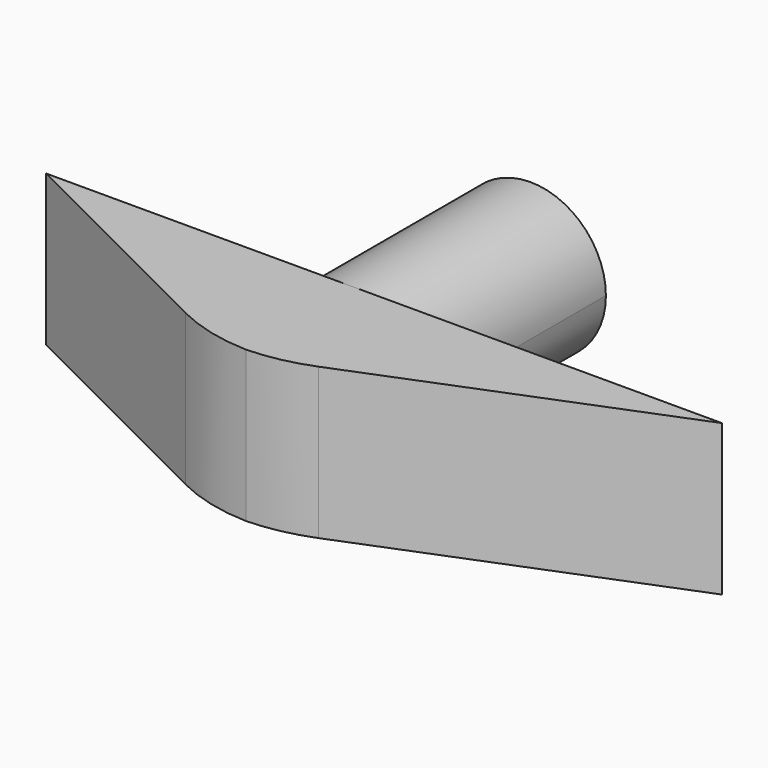
from build123d import *

# Parameters (mm, degrees)
F1_DEPTH    = 10
F2_DEPTH    = 6
F3_T1_DEPTH = 68.8558929709
F4_SIZE2    = 14.99999
F4_SIZE     = 5.99999
F5_T1_DEPTH = 16.1427191
F5_T3_DEPTH = 14.4032889904


# Not quite as in the source:
# - a fillet or chamfer that OpenCascade refuses, or shapes differently, is made with other operations: its cross-section is extruded or revolved along the edge and cut away or added
# - a fillet or chamfer is up to 0.001 mm smaller than in the source, because OpenCascade refuses the exact size


with BuildPart() as f1:
    # F0 (on Front) → F1 (new body)
    with BuildSketch(Plane.XZ):
        with BuildLine():
            ThreePointArc((2.15, -0.0081778196), (-3.4744734584, 2.4513486566), (-1.4615047685, -3.3479555451))
            Line((-1.4615047685, -3.3479555451), (-0.9384952315, -3.3479555451))
            ThreePointArc((-0.9384952315, -3.3479555451), (1.2595264762, -2.2826512779), (2.15, -0.0081778196))
        make_face()
    extrude(amount=-F1_DEPTH)


with BuildPart() as f2:
    # F0 (on Front) → F2 (new body)
    with BuildSketch(Plane.XZ):
        with BuildLine():
            Line((15.3, 3.3520444549), (-14.7, 3.3520444549))
            Line((-14.7, 3.3520444549), (-14.7, -3.3479555451))
            Line((-14.7, -3.3479555451), (-1.4615047685, -3.3479555451))
            ThreePointArc((-1.4615047685, -3.3479555451), (-3.4744734584, 2.4513486566), (2.15, -0.0081778196))
            ThreePointArc((2.15, -0.0081778196), (1.2595264762, -2.2826512779), (-0.9384952315, -3.3479555451))
            Line((-0.9384952315, -3.3479555451), (15.3, -3.3479555451))
            Line((15.3, -3.3479555451), (15.3, 3.3520444549))
        make_face()
        with BuildLine():
            ThreePointArc((2.15, -0.0081778196), (-3.4744734584, 2.4513486566), (-1.4615047685, -3.3479555451))
            Line((-1.4615047685, -3.3479555451), (-0.9384952315, -3.3479555451))
            ThreePointArc((-0.9384952315, -3.3479555451), (1.2595264762, -2.2826512779), (2.15, -0.0081778196))
        make_face()
    extrude(amount=F2_DEPTH)

    # F3: chamfer of 12 x 6 on 1 edges, made by hand

    # F3_s2 → F3_t1 (cut)
    with BuildSketch(Plane.XY.offset(-34.4259020306)):
        Polygon((-14.7, 0), (-2.7, -6), (-14.7, -6), align=None)
    extrude(amount=F3_T1_DEPTH, mode=Mode.SUBTRACT)

    # F4 (size 6 and 15 in the source; OpenCascade refuses exactly that, so slightly less here)
    f4_edges = [f2.edges().sort_by_distance(p)[0] for p in [
        (15.3, -6, 0.002044),
    ]]
    f4_side = f2.faces().sort_by_distance((15.3, -3, 0.002044))[0]
    chamfer(f4_edges, length=F4_SIZE, length2=F4_SIZE2, reference=f4_side)

    # F5: fillet of radius 8 on 2 edges, made by hand

    # F5_s2 → F5_t1 (cut)
    with BuildSketch(Plane.XY.offset(-8.0693150951)):
        with BuildLine():
            ThreePointArc((-0.81145618, -6), (-2.6494795444, -5.7859919157), (-4.389164944, -5.155417528))
            Line((-4.389164944, -5.155417528), (-2.7, -6))
            Line((-2.7, -6), (-0.81145618, -6))
        make_face()
    extrude(amount=F5_T1_DEPTH, mode=Mode.SUBTRACT)

    # F5_s4 → F5_t3 (cut)
    with BuildSketch(Plane.XY.offset(-7.1996000403)):
        with BuildLine():
            ThreePointArc((-1.2406477981, -6), (0.2722110167, -5.8556513547), (1.7304750514, -5.4278145516))
            Line((1.7304750514, -5.4278145516), (0.30001, -6))
            Line((0.30001, -6), (-1.2406477981, -6))
        make_face()
    extrude(amount=F5_T3_DEPTH, mode=Mode.SUBTRACT)


solid = Compound([f1.part, f2.part])
